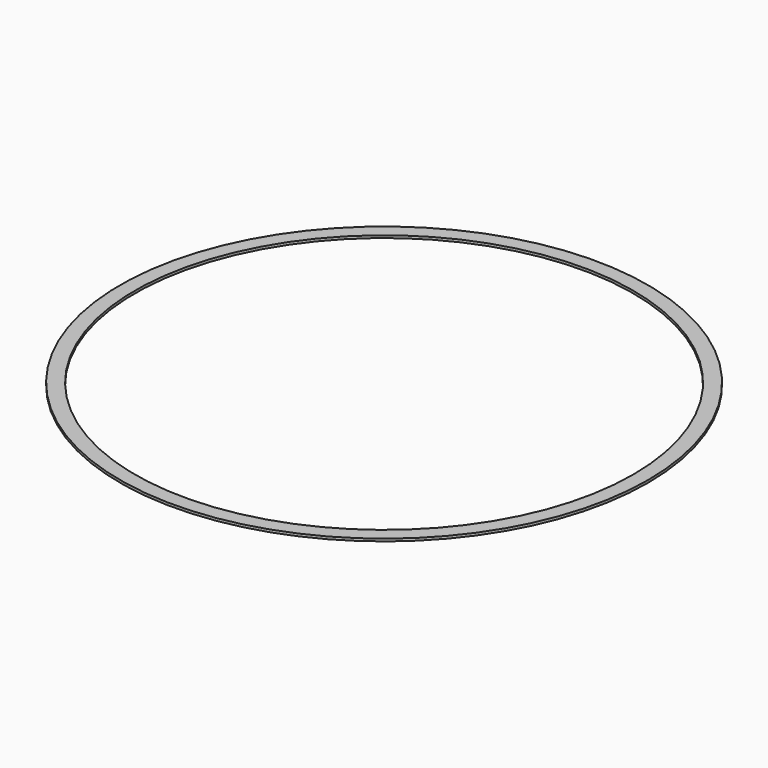
from build123d import *

# Parameters (mm, degrees)
F0_R     = 452.10095
F0_R_2   = 426.70095
F1_DEPTH = 4.2333333333


# Not quite as in the source:
# - a length typed as a fraction of an inch, garbled in the dataset ("3 / 203.2 mm" for 3/8 in), is restored


with BuildPart() as f1:
    # F0 (on Top) → F1 (new body)
    with BuildSketch(Plane.XY):
        Circle(F0_R)
        Circle(F0_R_2, mode=Mode.SUBTRACT)
    extrude(amount=F1_DEPTH)


solid = f1.part
